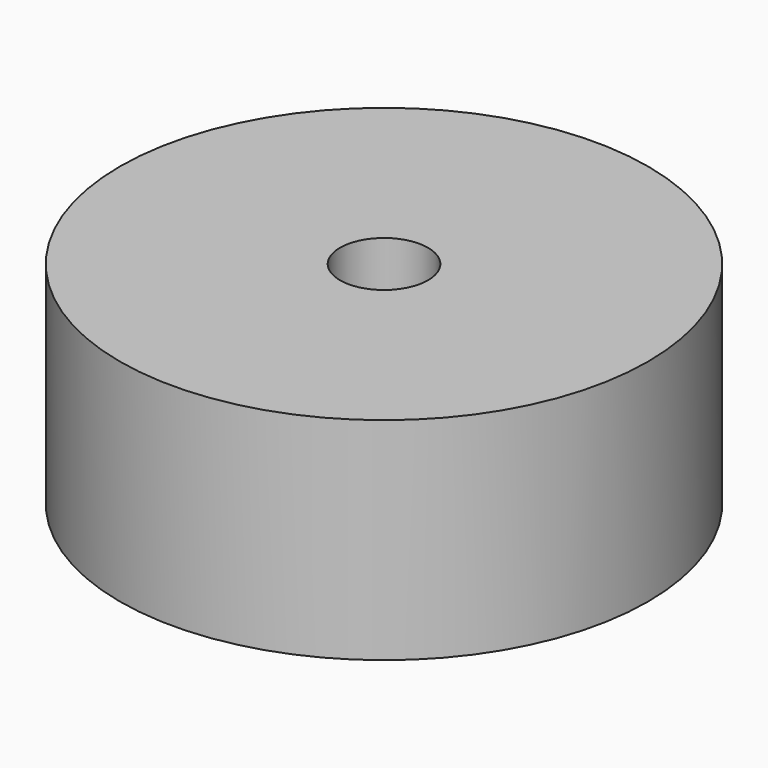
from build123d import *

# Parameters (mm, degrees)
F0_R     = 9.525
F0_R_2   = 1.5875
F1_DEPTH = 7.62


# Not quite as in the source:
# - the program builds the solid bodies; features that only make, move or delete a surface that nothing else refers to are left out


with BuildPart() as f1:
    # F0 (on Top) → F1 (new body)
    with BuildSketch(Plane.XY):
        Circle(F0_R)
        Circle(F0_R_2, mode=Mode.SUBTRACT)
    extrude(amount=F1_DEPTH)


solid = f1.part
